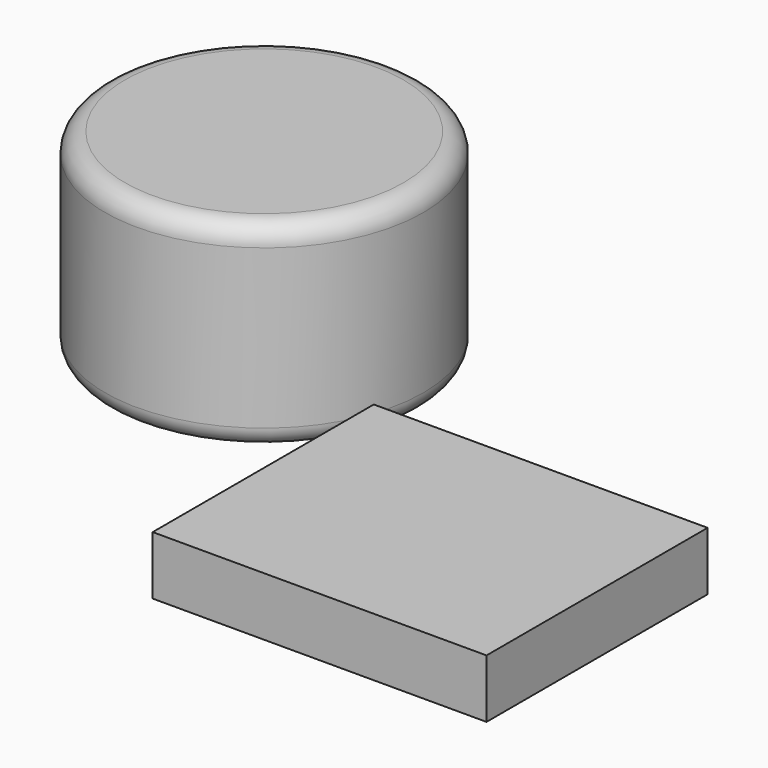
from build123d import *

# Parameters (mm, degrees)
F0_R     = 40.7744755984
F1_DEPTH = 25.4
F3_R     = 5.08
F4_R     = 5.08
F7_W     = 85.5231583118
F7_H     = 70.7953497767
F8_DEPTH = 15


with BuildPart() as f1:
    # F0 (on Top) → F1 (new body)
    with BuildSketch(Plane.XY):
        with Locations((-11.2624429166, 17.9966315627)):
            Circle(F0_R)
    extrude(amount=F1_DEPTH)

    # F2: F1 across plane


with BuildPart() as f1_1:
    add(f1.part)
    add(f1.part.mirror(Plane.XY))

    # F3
    f3_edges = [f1_1.edges().sort_by_distance(p)[0] for p in [
        (-52.036919, 17.996632, 25.4),
    ]]
    fillet(f3_edges, radius=F3_R)

    # F4
    f4_edges = [f1_1.edges().sort_by_distance(p)[0] for p in [
        (-52.036919, 17.996632, -25.4),
    ]]
    fillet(f4_edges, radius=F4_R)


with BuildPart() as f8:
    # F7 (on Top) → F8 (new body)
    with BuildSketch(Plane.XY):
        with Locations((110.0564450026, -80.5193148553)):
            Rectangle(F7_W, F7_H)
    extrude(amount=F8_DEPTH)


solid = Compound([f1_1.part, f8.part])
